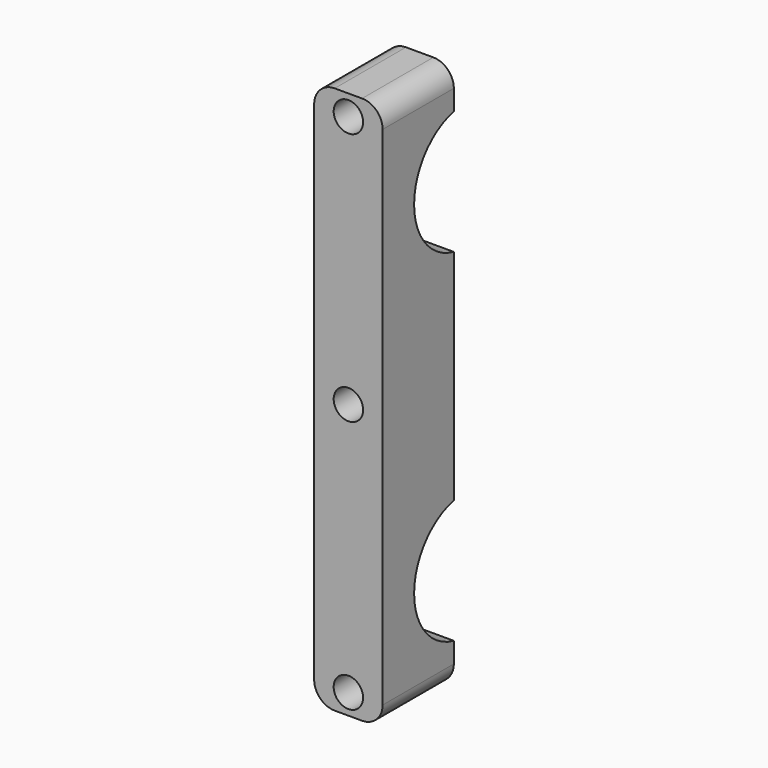
from build123d import *

# Parameters (mm, degrees)
F0_R     = 2.15
F1_DEPTH = 13
F3_DEPTH = 25


# Not quite as in the source:
# - a feature names something its author has since deleted; it is built from what else it names


with BuildPart() as f1:
    # F0 (on Front) → F1 (new body)
    with BuildSketch(Plane.XZ):
        with BuildLine():
            Line((2, 38.987471127), (-2, 38.987471127))
            ThreePointArc((-2, 38.987471127), (-4.1213203436, 38.1087914705), (-5, 35.987471127))
            Line((-5, 35.987471127), (-5, -38.012528873))
            ThreePointArc((-5, -38.012528873), (-4.1213203436, -40.1338492166), (-2, -41.012528873))
            Line((-2, -41.012528873), (2, -41.012528873))
            ThreePointArc((2, -41.012528873), (4.1213203436, -40.1338492166), (5, -38.012528873))
            Line((5, -38.012528873), (5, 35.987471127))
            ThreePointArc((5, 35.987471127), (4.1213203436, 38.1087914705), (2, 38.987471127))
        make_face()
        with Locations((0, -38.012528873)):
            Circle(F0_R, mode=Mode.SUBTRACT)
        with Locations((0, -1.012528873)):
            Circle(F0_R, mode=Mode.SUBTRACT)
        with Locations((0, 35.987471127)):
            Circle(F0_R, mode=Mode.SUBTRACT)
    extrude(amount=F1_DEPTH)

    # F2 (on face) → F3 (cut)
    with BuildSketch(Plane(origin=(-5, 0, 0), x_dir=(0, -1, 0), z_dir=(-1, 0, 0))):
        with BuildLine():
            ThreePointArc((0, 14.9562751929), (5.2132690231, 18.196853716), (7.25, 23.987471127))
            ThreePointArc((7.25, 23.987471127), (5.2132690231, 29.7780885379), (0, 33.0186670611))
            Line((0, 33.0186670611), (0, 23.987471127))
            Line((0, 23.987471127), (0, 14.9562751929))
        make_face()
        with BuildLine():
            ThreePointArc((7.25, -26.012528873), (5.2132690231, -20.2219114621), (0, -16.9813329389))
            Line((0, -16.9813329389), (0, -35.0437248071))
            ThreePointArc((0, -35.0437248071), (5.2132690231, -31.803146284), (7.25, -26.012528873))
        make_face()
    extrude(amount=-F3_DEPTH, mode=Mode.SUBTRACT)


solid = f1.part
